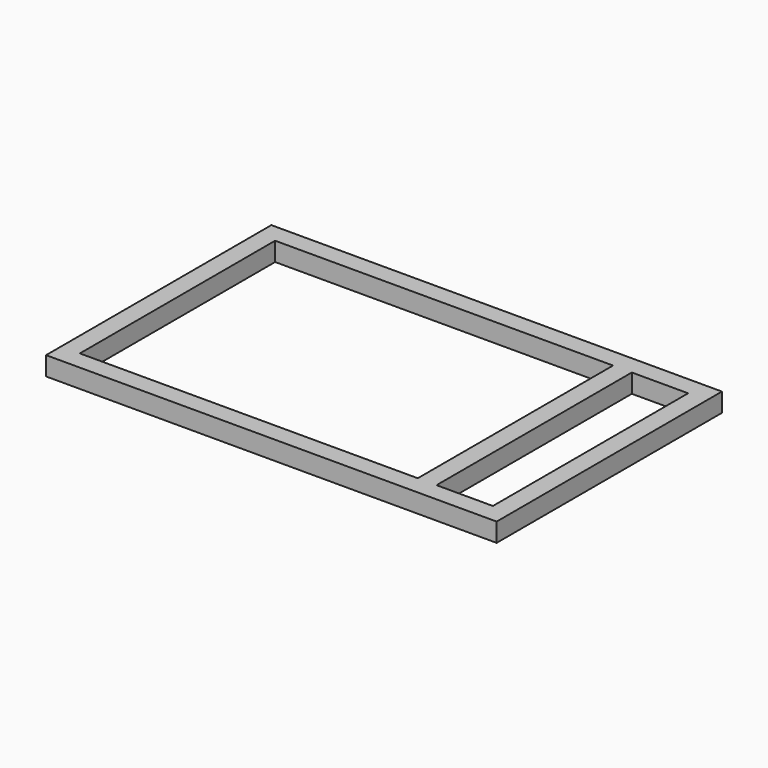
from build123d import *

# Parameters (mm, degrees)
F1_W     = 50.8
F1_H     = 50.8
F3_W     = 50.8
F3_H     = 50.8
F4_DEPTH = 660.4


with BuildPart() as f2:
    # F2: sweep along a path in F0
    with BuildLine(Plane.XY) as f2_path:
        Line((0, 0), (0, 762))
        Line((0, 762), (1219.2, 762))
        Line((1219.2, 762), (1219.2, 0))
        Line((1219.2, 0), (0, 0))
    # F1 (on Front) → F2 (sweep)
    with BuildSketch(Plane.XZ):
        with Locations((25.4, -25.4)):
            Rectangle(F1_W, F1_H)
    sweep(path=f2_path.line, transition=Transition.RIGHT)

    # F3 (on face) → F4 (join, through all)
    with BuildSketch(Plane.XZ.offset(-711.2)):
        with Locations((990.6, -25.4)):
            Rectangle(F3_W, F3_H)
    extrude(amount=F4_DEPTH)


solid = f2.part
